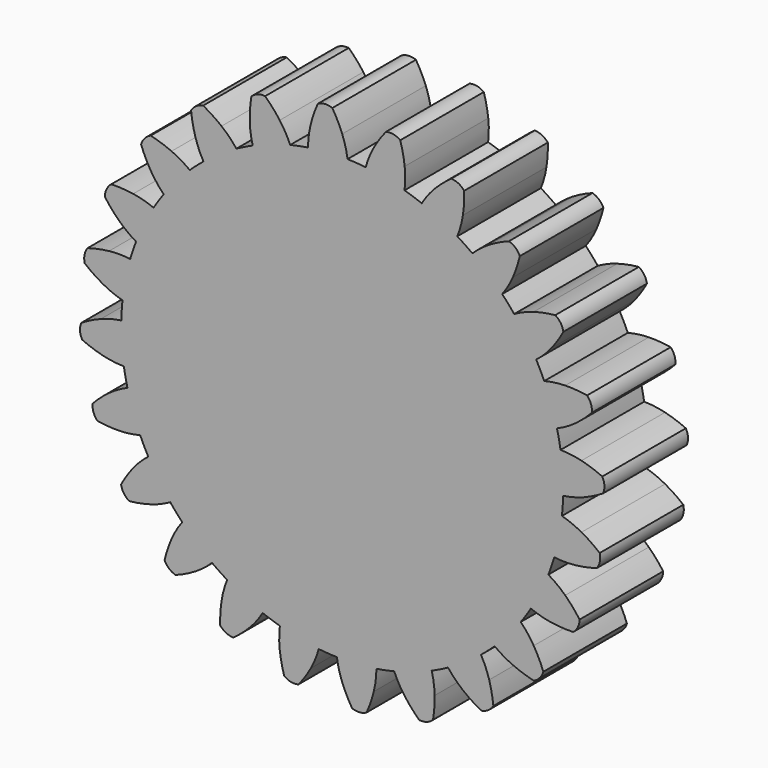
from build123d import *

# Parameters (mm, degrees)
F1_DEPTH        = 25.4
F1_COPIES_COUNT = 24


# Not quite as in the source:
# - a feature of the source that left no trace in its solid (it failed there, or was rolled back) is left out
# - a pattern or mirror of a feature is missing from the dataset's text; its kind, count and spacing are read off the source's solid


with BuildPart() as f1:
    # F0 (on Front) → F1 (new body)
    with BuildSketch(Plane.XZ):
        with BuildLine():
            ThreePointArc((-8.311718756, 53.0741101887), (-34.9244326919, -40.8194787099), (53.721, 0))
            ThreePointArc((53.721, 0), (38.4426942246, 37.524726538), (1.2981075836, 53.7053140546))
            ThreePointArc((1.2981075836, 53.7053140546), (-3.5209785571, 53.6054899334), (-8.311718756, 53.0741101887))
        make_face()
        with BuildLine():
            ThreePointArc((-8.311718756, 53.0741101887), (-3.5209785571, 53.6054899334), (1.2981075836, 53.7053140546))
            ThreePointArc((1.2981075836, 53.7053140546), (0.795324238, 56.2278713112), (0, 58.674))
            ThreePointArc((0, 58.674), (-1.0893912859, 61.1194533791), (-2.398474509, 63.45468714))
            ThreePointArc((-2.398474509, 63.45468714), (-4.1863086874, 63.734874996), (-5.9221335642, 63.22324204))
            ThreePointArc((-5.9221335642, 63.22324204), (-6.9145165038, 60.7368406838), (-7.6746780384, 58.1699028107))
            ThreePointArc((-7.6746780384, 58.1699028107), (-8.1432106678, 55.6407599953), (-8.311718756, 53.0741101887))
        make_face()
    extrude(amount=F1_DEPTH)

    # F1_copies: F1 ×24 about axis
    f1_copies_axis = Axis((0, 0, 0), (0, 1, 0))


with BuildPart() as f1_1:
    add(f1.part)
    for i in range(1, F1_COPIES_COUNT):
        add(f1.part.rotate(f1_copies_axis, i * 360 / F1_COPIES_COUNT))


solid = f1_1.part
